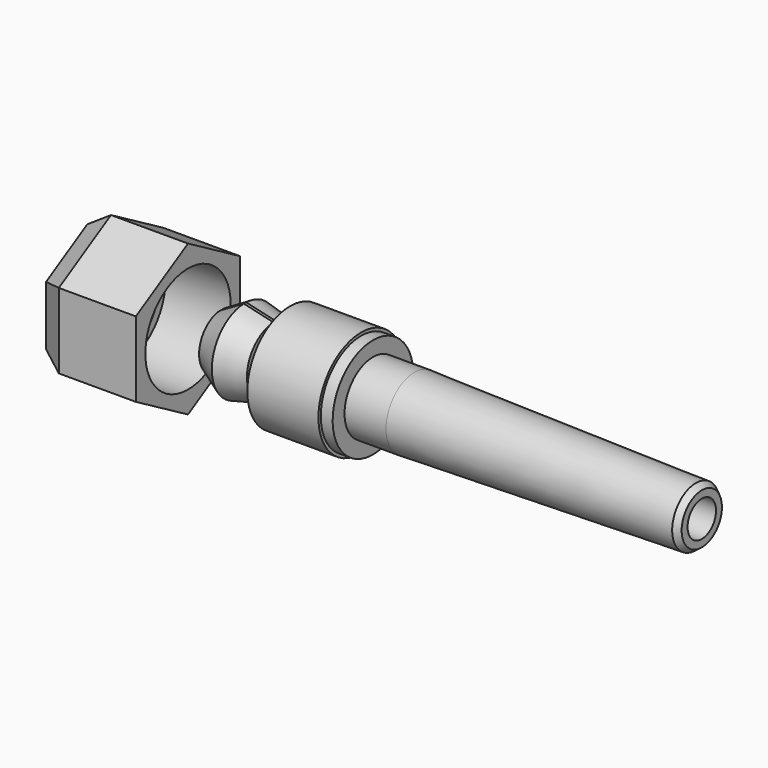
from build123d import *

# Parameters (mm, degrees)
F3_D         = 19.05
F3_DEPTH     = 47.625
F3_TIP       = 5.7231973962
F6_R         = 6.35
F7_DEPTH     = 44.45
F8_W         = 1.5875
F8_H         = 50.8
F9_DEPTH     = 50.8
F10_W        = 53.975
F10_H        = 88.9
F11_DEPTH    = 34.925
F13_DEPTH    = 53.975
F14_C1_SIZE2 = 7.3323484187
F14_C1_SIZE  = 12.7
F14_C2_SIZE2 = 7.3323484187
F14_C2_SIZE  = 12.7
F14_C3_SIZE2 = 12.7
F14_C3_SIZE  = 7.3323484187
F14_C4_SIZE2 = 12.7
F14_C4_SIZE  = 7.3323484187
F14_C5_SIZE2 = 12.7
F14_C5_SIZE  = 7.3323484187
F14_C6_SIZE2 = 12.7
F14_C6_SIZE  = 7.3323484187
F15_R        = 15.08125
F16_DEPTH    = 53.976
F17_R        = 28.575
F18_DEPTH    = 34.925


with BuildPart() as f1:
    # F0 (on Front) → F1 (revolve)
    with BuildSketch(Plane.XZ):
        Polygon((38.1, 26.9875), (38.1, 0), (44.45, 0), (44.45, 19.0246), (44.45, 26.9875), align=None)
        Polygon((31.75, 14.4980599318), (31.75, 0), (38.1, 0), (38.1, 26.9875), (38.1, 28.575), (0, 28.575), (0, 21.828125), align=None)
        Polygon((44.45, 19.0246), (44.45, 0), (217.4875, 0), (220.6625, 0), (220.6625, 13.49375), (217.4875, 15.875), (66.675, 19.0246), align=None)
    revolve(axis=Axis((130.96875, 0, 0), (1, 0, 0)))

    # F3
    with Locations(Plane.YZ.offset(220.6625)):
        with Locations((0, 0)):
            Hole(F3_D / 2, depth=F3_DEPTH)
            with Locations((0, 0, -(F3_DEPTH + F3_TIP / 2))):  # 118° drill point
                Cone(0, F3_D / 2, F3_TIP, mode=Mode.SUBTRACT)


with BuildPart() as f5:
    # F4 (on Front) → F5 (revolve)
    with BuildSketch(Plane.XZ):
        Polygon((-24.1045645936, 0), (-8.2295645936, 0), (-8.2295645936, 7.1290070594), (-8.2295645936, 18.5599674659), (-24.1045645936, 22.225), (-36.8045645936, 14.8926515813), (-36.8045645936, 0), align=None)
    revolve(axis=Axis((-30.4545645936, 0, 0), (-1, 0, 0)))

    # F6 (on face) → F7 (cut)
    with BuildSketch(Plane(origin=(-36.8045645936, 0, 0), x_dir=(0, -1, 0), z_dir=(-1, 0, 0))):
        Circle(F6_R)
    extrude(amount=-F7_DEPTH, mode=Mode.SUBTRACT)

    # F8 (on face) → F9 (cut)
    with BuildSketch(Plane(origin=(-36.8045645936, 0, 0), x_dir=(0, -1, 0), z_dir=(-1, 0, 0))):
        Rectangle(F8_W, F8_H)
    extrude(amount=-F9_DEPTH, mode=Mode.SUBTRACT)


with BuildPart() as f11:
    # F10 (on Front) → F11 (new body, symmetric)
    with BuildSketch(Plane.XZ):
        with Locations((-81.6434432337, 0)):
            Rectangle(F10_W, F10_H)
    extrude(amount=F11_DEPTH, both=True)

    # F12 (on face) → F13 (cut)
    with BuildSketch(Plane(origin=(-108.6309432337, 0, 0), x_dir=(0, -1, 0), z_dir=(-1, 0, 0))):
        Polygon((0, 40.3279163029), (34.925, 20.1639581514), (34.925, 44.45), (-34.925, 44.45), (-34.925, 20.1639581514), align=None)
        Polygon((34.925, -44.45), (34.925, -20.1639581514), (0, -40.3279163029), (-34.925, -20.1639581514), (-34.925, -44.45), align=None)
    extrude(amount=-F13_DEPTH, mode=Mode.SUBTRACT)

    # F14: chamfer of 12.7 x 7.3323484187 on 6 edges, made by hand

    # F14_c1
    f14_c1_edges = [f11.edges().sort_by_distance(p)[0] for p in [
        (-108.6309432337, 34.925, 0),
    ]]
    f14_c1_side = f11.faces().sort_by_distance((-108.4842962653, 34.925, 0))[0]
    chamfer(f14_c1_edges, length=F14_C1_SIZE, length2=F14_C1_SIZE2, reference=f14_c1_side)

    # F14_c2
    f14_c2_edges = [f11.edges().sort_by_distance(p)[0] for p in [
        (-108.6309432337, 13.7963257906, -32.3626038938),
    ]]
    f14_c2_side = f11.faces().sort_by_distance((-108.4842962653, 13.7963257906, -32.3626038938))[0]
    chamfer(f14_c2_edges, length=F14_C2_SIZE, length2=F14_C2_SIZE2, reference=f14_c2_side)

    # F14_c3
    f14_c3_edges = [f11.edges().sort_by_distance(p)[0] for p in [
        (-108.6309432337, 13.7963257906, 32.3626038938),
    ]]
    f14_c3_side = f11.faces().sort_by_distance((-108.6309432337, 13.7230023065, 32.2356038938))[0]
    chamfer(f14_c3_edges, length=F14_C3_SIZE, length2=F14_C3_SIZE2, reference=f14_c3_side)

    # F14_c4
    f14_c4_edges = [f11.edges().sort_by_distance(p)[0] for p in [
        (-108.6309432337, -21.1286742094, 28.1292705605),
    ]]
    f14_c4_side = f11.faces().sort_by_distance((-108.6309432337, -21.0553507252, 28.0022705605))[0]
    chamfer(f14_c4_edges, length=F14_C4_SIZE, length2=F14_C4_SIZE2, reference=f14_c4_side)

    # F14_c5
    f14_c5_edges = [f11.edges().sort_by_distance(p)[0] for p in [
        (-108.6309432337, -34.925, -4.2333333333),
    ]]
    f14_c5_side = f11.faces().sort_by_distance((-108.6309432337, -34.7783530316, -4.2333333333))[0]
    chamfer(f14_c5_edges, length=F14_C5_SIZE, length2=F14_C5_SIZE2, reference=f14_c5_side)

    # F14_c6
    f14_c6_edges = [f11.edges().sort_by_distance(p)[0] for p in [
        (-108.6309432337, -17.4625, -30.2459372272),
    ]]
    f14_c6_side = f11.faces().sort_by_distance((-108.6309432337, -17.3891765158, -30.1189372272))[0]
    chamfer(f14_c6_edges, length=F14_C6_SIZE, length2=F14_C6_SIZE2, reference=f14_c6_side)

    # F15 (on face) → F16 (cut, through all)
    with BuildSketch(Plane.YZ.offset(-54.6559432337)):
        Circle(F15_R)
    extrude(amount=-F16_DEPTH, mode=Mode.SUBTRACT)

    # F17 (on face) → F18 (cut)
    with BuildSketch(Plane.YZ.offset(-54.6559432337)):
        Circle(F17_R)
    extrude(amount=-F18_DEPTH, mode=Mode.SUBTRACT)

    # F19 (on Front) → F20 (revolve, cut)
    with BuildSketch(Plane.XZ):
        Polygon((-92.7559432337, 15.08125), (-105.4559432337, 15.08125), (-105.4559432337, 0), (-92.7559432337, 0), (-87.1003866196, 0), (-87.1003866196, 15.08125), align=None)
        Polygon((-97.1985902505, 19.8486349676), (-105.4559432337, 15.08125), (-92.7559432337, 15.08125), (-92.7559432337, 22.4135984187), align=None)
        Polygon((-92.7559432337, 22.4135984187), (-92.7559432337, 15.08125), (-87.1003866196, 15.08125), (-87.1003866196, 22.4286857992), (-87.1003866196, 25.6788355523), align=None)
    revolve(axis=Axis((-96.2781649266, 0, 0), (-1, 0, 0)), mode=Mode.SUBTRACT)


solid = Compound([f1.part, f5.part, f11.part])
